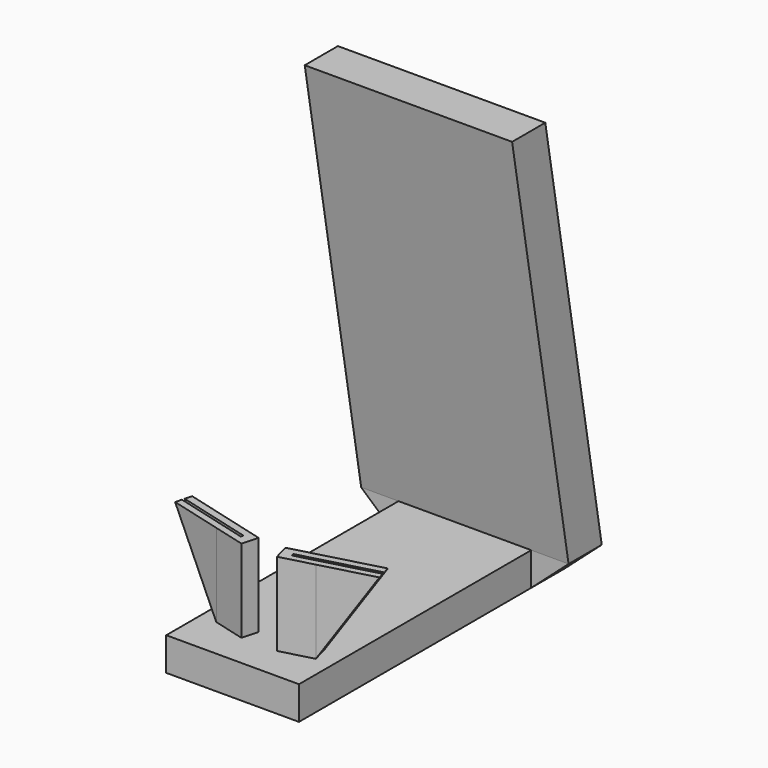
from build123d import *

# Parameters (mm, degrees)
F1_DEPTH  = 40
F4_DEPTH  = 62.5
F6_DEPTH  = 12.5
F8_DEPTH  = 25
F10_DEPTH = 5
F12_DEPTH = 15


# Not quite as in the source:
# - a pattern or mirror of a feature is missing from the dataset's text; its kind, count and spacing are read off the source's solid


with BuildPart() as f1:
    # F0 (on Right) → F1 (new body)
    with BuildSketch(Plane.YZ):
        Polygon((-57.0501919146, 0), (0, 0), (42.9498080854, 0), (42.9498080854, 10), (-57.0501919146, 10), align=None)
    extrude(amount=F1_DEPTH)

    # F3 (on offset) → F4 (join)
    with BuildSketch(Plane.YZ.offset(51.25)):
        Polygon((9.1779063212, 130.638949744), (30.4498080854, 10), (42.9498080854, 10), (21.6779063212, 130.638949744), align=None)
    extrude(amount=-F4_DEPTH)

    # F5 (on face) → F6 (join)
    with BuildSketch(Plane(origin=(0, 42.9498080854, 0), x_dir=(-1, 0, 0), z_dir=(0, 1, 0))):
        Polygon((11.25, 10), (0, 10), (0, 0), align=None)
        Polygon((-40, 0), (-40, 10), (-51.25, 10), align=None)
    extrude(amount=-F6_DEPTH)

    # F7 (on face) → F8 (join)
    with BuildSketch(Plane.XY.offset(10)):
        Polygon((15.9533534884, -42.2205627832), (6.2940952255, -39.6323723322), (5, -44.4620014636), (14.6592582629, -47.0501919146), align=None)
        Polygon((33.7059047745, -39.6323723322), (24.0466465116, -42.2205627832), (25.3407417371, -47.0501919146), (35, -44.4620014636), align=None)
    extrude(amount=F8_DEPTH)

    # F9 (on face) → F10 (join)
    with BuildSketch(Plane(origin=(-9.4864686499, -35.4039829857, 0), x_dir=(-0.9659258263, 0.2588190451, 0), z_dir=(0.2588190451, 0.9659258263, 0))):
        Polygon((-16.3372418936, 35), (-16.3372418936, 10), (0, 35), align=None)
    f10 = extrude(amount=-F10_DEPTH)

    # F10_copies: F10 across plane
    add(f10.mirror(Plane(origin=(20, 0, 0), x_dir=(0, 0, 1), z_dir=(1, 0, 0))))

    # F11 (on face) → F12 (cut)
    with BuildSketch(Plane.XY.offset(35)):
        Polygon((12.2791188742, -44.3418831268), (12.4861741103, -43.5691424657), (-10.0558705491, -37.5290198035), (-10.2629257852, -38.3017604645), align=None)
    f12 = extrude(amount=-F12_DEPTH, mode=Mode.SUBTRACT)

    # F12_copies: F12 across plane
    add(f12.mirror(Plane(origin=(20, 0, 0), x_dir=(0, 0, 1), z_dir=(1, 0, 0))), mode=Mode.SUBTRACT)


solid = f1.part
